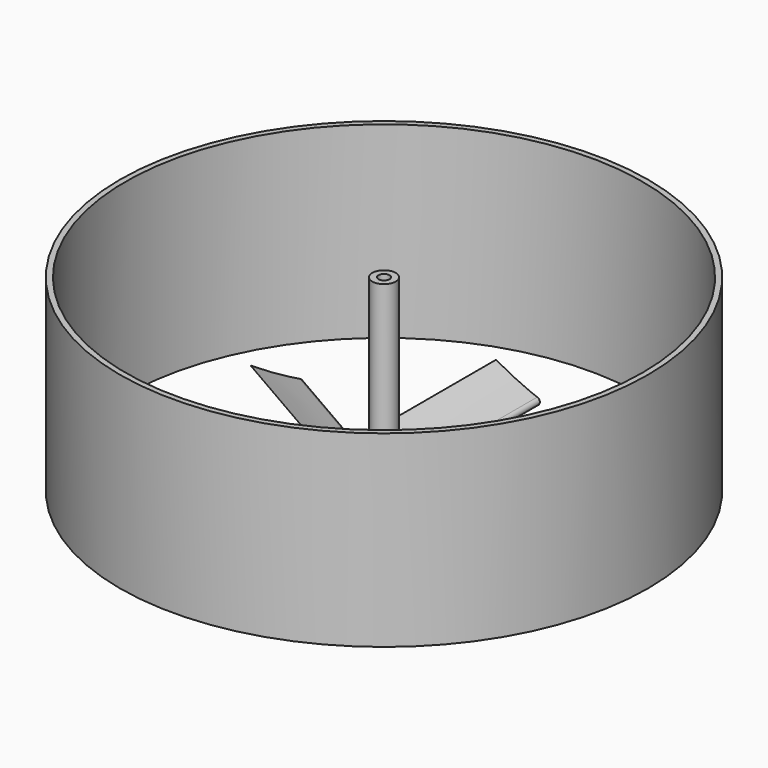
from build123d import *

# Parameters (mm, degrees)
F1_DEPTH        = 50.8
F1_COPIES_COUNT = 6
F4_R            = 3.175
F5_DEPTH        = 50.8
F6_W            = 254
F6_H            = 23.0000000447
F10_R           = 71.35
F10_R_2         = 69.85
F11_DEPTH       = 50.8
F13_D           = 3
F13_DEPTH       = 20
F13_TIP         = 0.9012909285


# Not quite as in the source:
# - a pattern or mirror of a feature is missing from the dataset's text; its kind, count and spacing are read off the source's solid


with BuildPart() as f1:
    # F0 (on Front) → F1 (new body)
    with BuildSketch(Plane.XZ):
        with BuildLine():
            ThreePointArc((-0.7517356134, 1.875386318), (-1.3892537051, 0.5314844421), (0, 0))
            add(Edge.make_bspline(
                [(0, 0), (0.8457416774, 0.417742316), (2.6483568704, 1.4876087408), (7.3696031318, 4.6379577961), (9.4162562728, 6.3605664752), (10.3752381482, 7.1448470762)],
                knots=[0, 0, 0, 0, 0.2848386948, 0.6737205223, 1, 1, 1, 1], degree=3))
            add(Edge.make_bspline(
                [(-0.7517356134, 1.875386318), (0.3878314468, 2.232497367), (2.3095512481, 3.1741762509), (6.2154828863, 4.8060582002), (8.9039475225, 6.3321645003), (10.3752381482, 7.1448470762)],
                knots=[0, 0, 0, 0, 0.3013068645, 0.6364852042, 1, 1, 1, 1], degree=3))
        make_face()
    extrude(amount=F1_DEPTH)

    # F1_copies: F1 ×6 about axis
    f1_copies_axis = Axis((0, 0, 0), (0, 0, 1))


with BuildPart() as f1_1:
    add(f1.part)
    for i in range(1, F1_COPIES_COUNT):
        add(f1.part.rotate(f1_copies_axis, i * 360 / F1_COPIES_COUNT))

    # F2 (on Front) → F3 (revolve, cut)
    with BuildSketch(Plane.XZ):
        Polygon((0, 7.7916895971), (0, 2.1290599834), (20.2574506402, 7.7916895971), align=None)
    revolve(axis=Axis((0, 0, 14.8271257058), (0, 0, 1)), mode=Mode.SUBTRACT)

    # F4 (on Top) → F5 (join)
    with BuildSketch(Plane.XY):
        Circle(F4_R)
    extrude(amount=F5_DEPTH)

    # F6 (on Right) → F7 (revolve, cut)
    with BuildSketch(Plane.YZ):
        with Locations((-127, -11.5000000224)):
            Rectangle(F6_W, F6_H)
    revolve(axis=Axis((0, 0, 14.8271257058), (0, 0, 1)), mode=Mode.SUBTRACT)

    # F8 (on Right) → F9 (revolve)
    with BuildSketch(Plane.YZ):
        with BuildLine():
            Line((-9.6497299307, 3.9679169684), (-11.5, 0))
            Line((-11.5, 0), (-1.5, 0))
            Line((-1.5, 0), (-1.5, 12.5))
            Line((-1.5, 12.5), (-3, 12.5))
            add(Edge.make_bspline(
                [(-3, 12.5), (-3.3669461986, 10.9728953245), (-4.4961179612, 8.2898794508), (-6.8188407016, 5.484266906), (-8.6877416586, 4.4783924105), (-9.6497299307, 3.9679169684)],
                knots=[0, 0, 0, 0, 0.3672608642, 0.6920053155, 1, 1, 1, 1], degree=3))
        make_face()
    revolve(axis=Axis((0, 0, 14.8271257058), (0, 0, 1)))

    # F13
    with Locations(Plane.XY.offset(50.8)):
        with Locations((0, 0)):
            Hole(F13_D / 2, depth=F13_DEPTH)
            with Locations((0, 0, -(F13_DEPTH + F13_TIP / 2))):  # 118° drill point
                Cone(0, F13_D / 2, F13_TIP, mode=Mode.SUBTRACT)


with BuildPart() as f11:
    # F10 (on Top) → F11 (new body)
    with BuildSketch(Plane.XY):
        Circle(F10_R)
        Circle(F10_R_2, mode=Mode.SUBTRACT)
    extrude(amount=F11_DEPTH)


solid = Compound([f1_1.part, f11.part])
